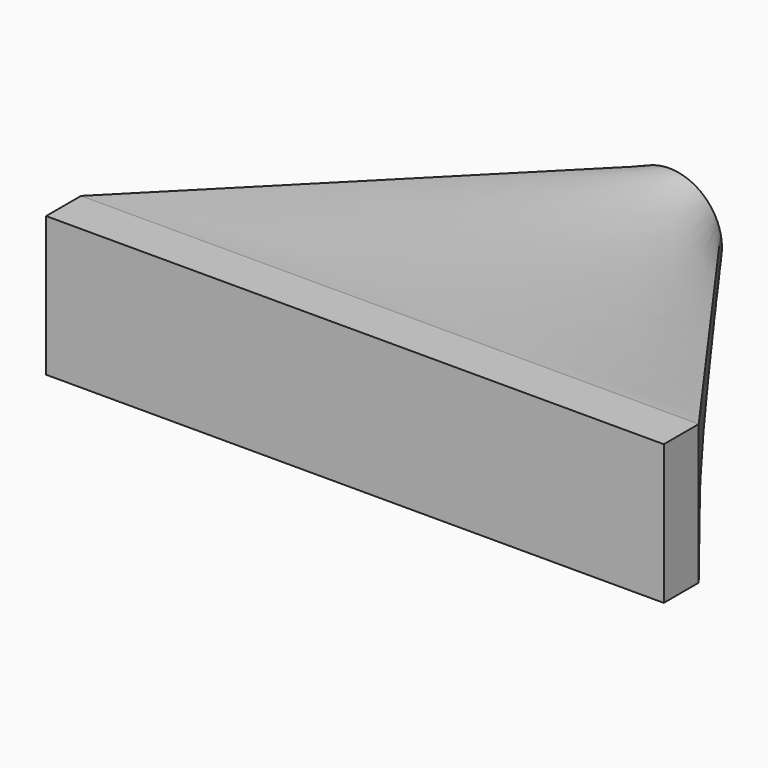
from build123d import *

# Parameters (mm, degrees)
F2_W     = 14.15
F2_H     = 3.2
F4_W     = 14.15
F4_H     = 3.2
F5_DEPTH = 1


# Not quite as in the source:
# - the arcs of a loft's sections are written as splines that run evenly, so that the points pair up as in the source's solid


with BuildPart() as f3:
    # F2 (on offset) → F3 section 0
    with BuildSketch(Plane.XZ.offset(8)):
        Rectangle(F2_W, F2_H)
    # F0 (on Front) → F3 section 1
    with BuildSketch(Plane.XZ):
        with BuildLine():
            add(Edge.make_bspline(
                [(1.1777584175, 0.2663481933), (1.1428935205, 0.4205164097), (1.0773884422, 0.5676916369), (0.8949712684, 0.8258729192), (0.7781309462, 0.9367773911), (0.5107977536, 1.1054977634), (0.3604100674, 1.1632472795), (0.0488599113, 1.2168205944), (-0.112179977, 1.2126233144), (-0.2663481933, 1.1777584175)],
                knots=[0, 0, 0, 0, 0.25, 0.25, 0.5, 0.5, 0.75, 0.75, 1, 1, 1, 1], degree=3))
            add(Edge.make_bspline(
                [(-0.2663481933, 1.1777584175), (-0.4205164097, 1.1428935205), (-0.5676916369, 1.0773884422), (-0.8258729192, 0.8949712684), (-0.9367773911, 0.7781309462), (-1.1054977634, 0.5107977536), (-1.1632472795, 0.3604100674), (-1.2168205944, 0.0488599113), (-1.2126233144, -0.112179977), (-1.1777584175, -0.2663481933)],
                knots=[0, 0, 0, 0, 0.25, 0.25, 0.5, 0.5, 0.75, 0.75, 1, 1, 1, 1], degree=3))
            add(Edge.make_bspline(
                [(-1.1777584175, -0.2663481933), (-1.1428935205, -0.4205164097), (-1.0773884422, -0.5676916369), (-0.8949712684, -0.8258729192), (-0.7781309462, -0.9367773911), (-0.5107977536, -1.1054977634), (-0.3604100674, -1.1632472795), (-0.0488599113, -1.2168205944), (0.112179977, -1.2126233144), (0.2663481933, -1.1777584175)],
                knots=[0, 0, 0, 0, 0.25, 0.25, 0.5, 0.5, 0.75, 0.75, 1, 1, 1, 1], degree=3))
            add(Edge.make_bspline(
                [(0.2663481933, -1.1777584175), (0.4205164097, -1.1428935205), (0.5676916369, -1.0773884422), (0.8258729192, -0.8949712684), (0.9367773911, -0.7781309462), (1.1054977634, -0.5107977536), (1.1632472795, -0.3604100674), (1.2168205944, -0.0488599113), (1.2126233144, 0.112179977), (1.1777584175, 0.2663481933)],
                knots=[0, 0, 0, 0, 0.25, 0.25, 0.5, 0.5, 0.75, 0.75, 1, 1, 1, 1], degree=3))
        make_face()
    loft(ruled=True)

    # F4 (on face) → F5 (join)
    with BuildSketch(Plane.XZ.offset(8)):
        Rectangle(F4_W, F4_H)
    extrude(amount=F5_DEPTH)


solid = f3.part
